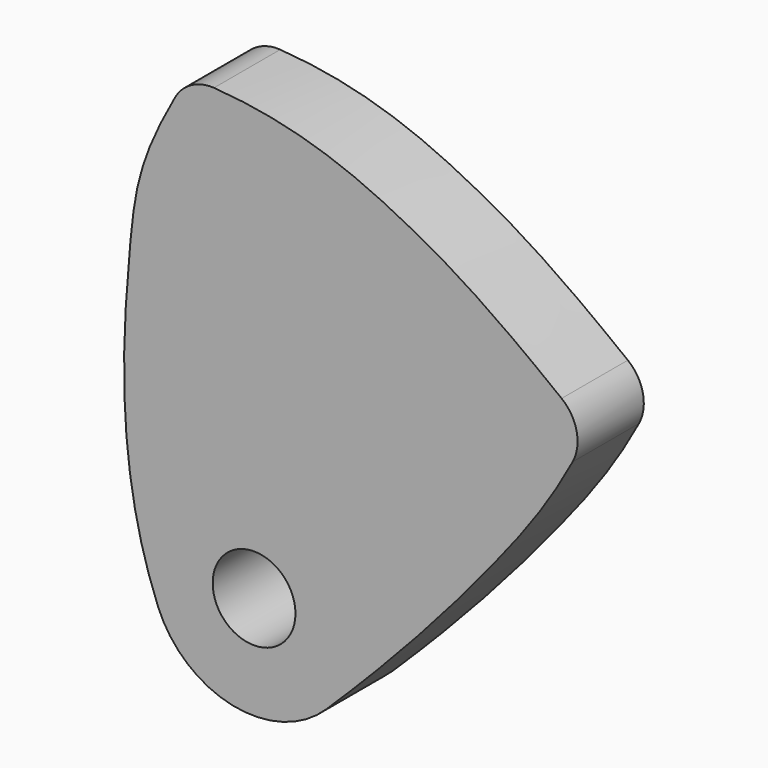
from build123d import *

# Parameters (mm, degrees)
F0_R     = 3.175
F1_DEPTH = 6.35


with BuildPart() as f1:
    # F0 (on Front) → F1 (new body)
    with BuildSketch(Plane.XZ):
        with BuildLine():
            add(Edge.make_bspline(
                [(-6.0602840723, 31.8534711944), (-8.9123209928, 26.7616721507), (-9.5678060072, 21.1194401062), (-10.7354209084, 5.442497338), (-7.3669134372, -2.9550791291)],
                knots=[0, 0, 0, 0, 0.4184743156, 1, 1, 1, 1], degree=3))
            ThreePointArc((-7.3669134372, -2.9550791291), (-1.63587801, -7.7670978741), (5.5491886165, -5.6754217419))
            add(Edge.make_bspline(
                [(24.4385115585, 17.1715788698), (22.5209788834, 13.5742014085), (17.275688011, 6.7190147021), (11.0943717174, -0.2535749894), (5.5491886165, -5.6754217419)],
                knots=[0.1380846356, 0.1380846356, 0.1380846356, 0.1380846356, 0.4828720967, 1, 1, 1, 1], degree=3))
            ThreePointArc((24.4385115585, 17.1715788698), (24.7420563147, 19.326379645), (23.5868786889, 21.1705245559))
            add(Edge.make_bspline(
                [(-3.074806905, 33.4695786248), (3.1958280854, 33.0431476028), (12.0935678521, 29.2874679133), (18.4108124786, 25.1994105978), (23.5868786889, 21.1705245559)],
                knots=[0, 0, 0, 0, 0.5068320595, 1, 1, 1, 1], degree=3))
            ThreePointArc((-3.074806905, 33.4695786248), (-4.8016804973, 33.0940485831), (-6.0602840723, 31.8534711944))
        make_face()
        Circle(F0_R, mode=Mode.SUBTRACT)
    extrude(amount=F1_DEPTH)


solid = f1.part
